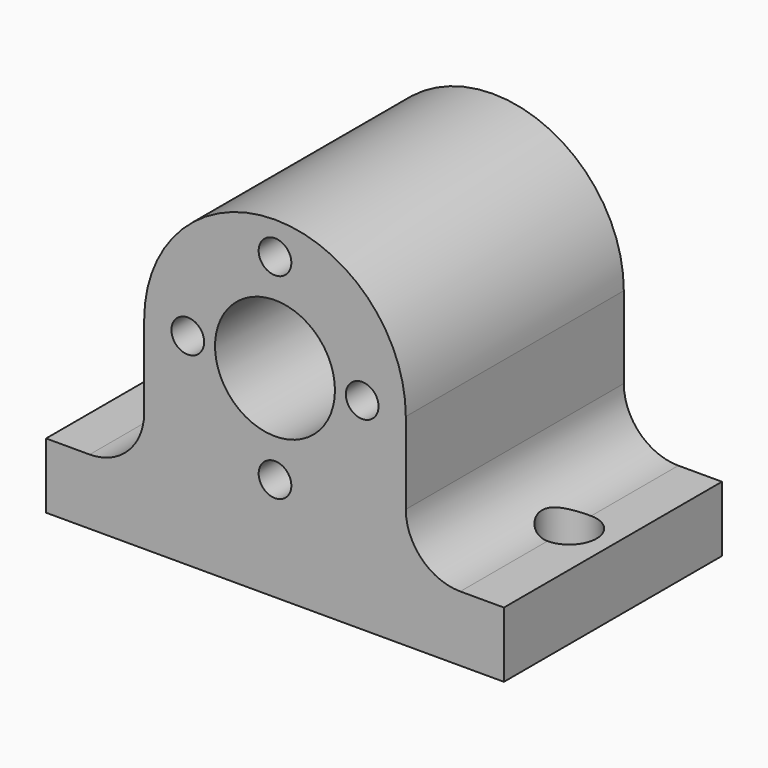
from build123d import *

# Parameters (mm, degrees)
F0_R         = 1.5
F0_R_2       = 5.5
F1_DEPTH     = 25
F2_R         = 2.5
F3_DEPTH     = 6.001
F4_T4_DEPTH  = 25
F4_S5_R      = 2.5
F4_T6_DEPTH  = 14
F4_T10_DEPTH = 25
F4_S11_R     = 2.5
F4_T12_DEPTH = 14


# Not quite as in the source:
# - a fillet or chamfer that OpenCascade refuses, or shapes differently, is made with other operations: its cross-section is extruded or revolved along the edge and cut away or added
# - a feature names something its author has since deleted; it is built from what else it names


with BuildPart() as f1:
    # F0 (on Front) → F1 (new body)
    with BuildSketch(Plane.XZ):
        with BuildLine():
            ThreePointArc((-12, 0), (0, -12), (12, 0))
            ThreePointArc((12, 0), (0, 12), (-12, 0))
        make_face()
        with Locations((0, -9)):
            Circle(F0_R, mode=Mode.SUBTRACT)
        with Locations((-8, 0)):
            Circle(F0_R, mode=Mode.SUBTRACT)
        Circle(F0_R_2, mode=Mode.SUBTRACT)
        with Locations((8, 0)):
            Circle(F0_R, mode=Mode.SUBTRACT)
        with Locations((0, 9)):
            Circle(F0_R, mode=Mode.SUBTRACT)
        with BuildLine():
            Line((12, -12.5), (12, 0))
            ThreePointArc((12, 0), (0, -12), (-12, 0))
            Line((-12, 0), (-12, -12.5))
            Line((-12, -12.5), (-21, -12.5))
            Line((-21, -12.5), (-21, -18.5))
            Line((-21, -18.5), (21, -18.5))
            Line((21, -18.5), (21, -12.5))
            Line((21, -12.5), (12, -12.5))
        make_face()
    extrude(amount=F1_DEPTH)

    # F2 (on face) → F3 (cut, through all)
    with BuildSketch(Plane.XY.offset(-12.5)):
        with Locations((17.000001, -12.5)):
            Circle(F2_R)
        with Locations((-17.000001, -12.5)):
            Circle(F2_R)
    extrude(amount=-F3_DEPTH, mode=Mode.SUBTRACT)

    # F4: fillet of radius 5 on 2 edges, made by hand


with BuildPart() as f4_tool2:
    # F4_s3 → F4_t4 (new body)
    with BuildSketch(Plane.XZ):
        with BuildLine():
            ThreePointArc((12, -7.5), (13.464466, -11.035534), (17, -12.5))
            Line((17, -12.5), (12, -12.5))
            Line((12, -12.5), (12, -7.5))
        make_face()
    extrude(amount=F4_T4_DEPTH)

    # F4_s5 → F4_t6 (cut, symmetric)
    with BuildSketch(Plane.XY.offset(-10)):
        with Locations((17.000001, -12.5)):
            Circle(F4_S5_R)
    extrude(amount=F4_T6_DEPTH, both=True, mode=Mode.SUBTRACT)


with BuildPart() as f1_1:
    add(f1.part)

    # F4_t1: union F4_tool2
    add(f4_tool2.part)


with BuildPart() as f4_tool8:
    # F4_s9 → F4_t10 (new body)
    with BuildSketch(Plane.XZ):
        with BuildLine():
            ThreePointArc((-12, -7.5), (-13.464466, -11.035534), (-17, -12.5))
            Line((-17, -12.5), (-12, -12.5))
            Line((-12, -12.5), (-12, -7.5))
        make_face()
    extrude(amount=F4_T10_DEPTH)

    # F4_s11 → F4_t12 (cut, symmetric)
    with BuildSketch(Plane.XY.offset(-10)):
        with Locations((-17.000001, -12.5)):
            Circle(F4_S11_R)
    extrude(amount=F4_T12_DEPTH, both=True, mode=Mode.SUBTRACT)


with BuildPart() as f1_2:
    add(f1_1.part)

    # F4_t7: union F4_tool8
    add(f4_tool8.part)


solid = f1_2.part
